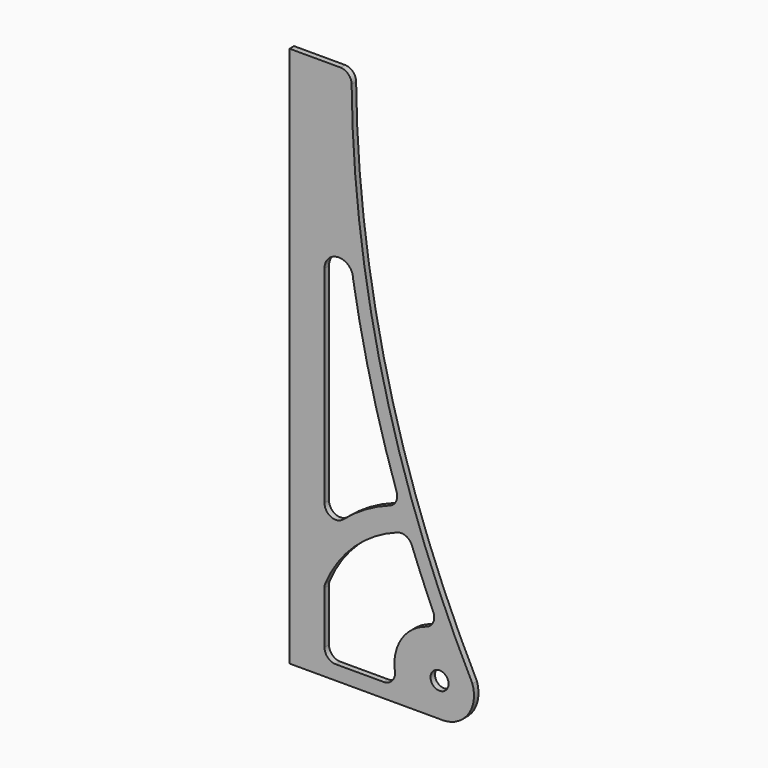
from build123d import *

# Parameters (mm, degrees)
F0_R     = 9.6
F1_DEPTH = 6


# Not quite as in the source:
# - ends of sketch curves that miss each other by under 0.0002 mm in the source are joined


with BuildPart() as f1:
    # F0 (on Front) → F1 (new body)
    with BuildSketch(Plane.XZ):
        with BuildLine():
            Line((-98.148557, 288.055726), (-98.148557, -287.944274))
            Line((-98.148557, -287.944274), (61.451443, -287.944274))
            ThreePointArc((61.451443, -287.944274), (90.8786929022, -275.1012880869), (96.4420569386, -243.4792343499))
            ThreePointArc((96.4420569386, -243.4792343499), (1.8673791595, 8.8528531517), (-32.087896312, 276.178294007))
            ThreePointArc((-32.087896312, 276.178294007), (-35.6454351808, 284.5842316136), (-44.087271, 288.055726))
            Line((-44.087271, 288.055726), (-98.148557, 288.055726))
        make_face()
        with BuildLine():
            ThreePointArc((-59.9885571325, -200.2110509435), (-29.1876571231, -155.9830655412), (16.7239738658, -127.7530766274))
            ThreePointArc((16.7239738658, -127.7530766274), (25.780399848, -128.1300293864), (31.9895542757, -134.7336148939))
            ThreePointArc((31.9895542757, -134.7336148939), (43.0295184538, -162.3758186302), (54.7647919037, -189.7300795987))
            ThreePointArc((54.7647919037, -189.7300795987), (54.7194507021, -199.5712496832), (47.3282871338, -206.0690474345))
            ThreePointArc((47.3282871338, -206.0690474345), (20.885121351, -226.2854831503), (13.9494494618, -258.8406940781))
            ThreePointArc((13.9494494618, -258.8406940781), (11.1483451659, -268.4168923847), (2.073951, -272.564799))
            Line((2.073951, -272.564799), (-48.948557, -272.564799))
            ThreePointArc((-48.948557, -272.564799), (-57.4338383742, -269.0500803742), (-60.948557, -260.564799))
            Line((-60.948557, -260.564799), (-60.948557, -204.914071))
            ThreePointArc((-60.948557, -204.914071), (-60.7061077935, -202.514071138), (-59.9885571325, -200.2110509435))
        make_face(mode=Mode.SUBTRACT)
        with BuildLine():
            ThreePointArc((-31.3094104055, 99.2474937685), (-30.7081992917, 96.8404508863), (-30.506005, 94.367714))
            ThreePointArc((-30.506005, 94.367714), (-11.0707369719, 1.2206915156), (15.8236014105, -90.0524808608))
            ThreePointArc((15.8236014105, -90.0524808608), (15.2706893662, -99.1138555668), (8.5302342503, -105.1950136941))
            ThreePointArc((8.5302342503, -105.1950136941), (-17.6222584193, -117.4699279564), (-41.0628425771, -134.3567693381))
            ThreePointArc((-41.0628425771, -134.3567693381), (-53.9170288848, -136.2346849428), (-60.948557, -125.311577))
            Line((-60.948557, -125.311577), (-60.948557, 94.367714))
            ThreePointArc((-60.948557, 94.367714), (-48.2000178863, 109.3867957083), (-31.3094104055, 99.2474937685))
        make_face(mode=Mode.SUBTRACT)
        with Locations((61.451443, -251.944274)):
            Circle(F0_R, mode=Mode.SUBTRACT)
    extrude(amount=F1_DEPTH)


solid = f1.part
